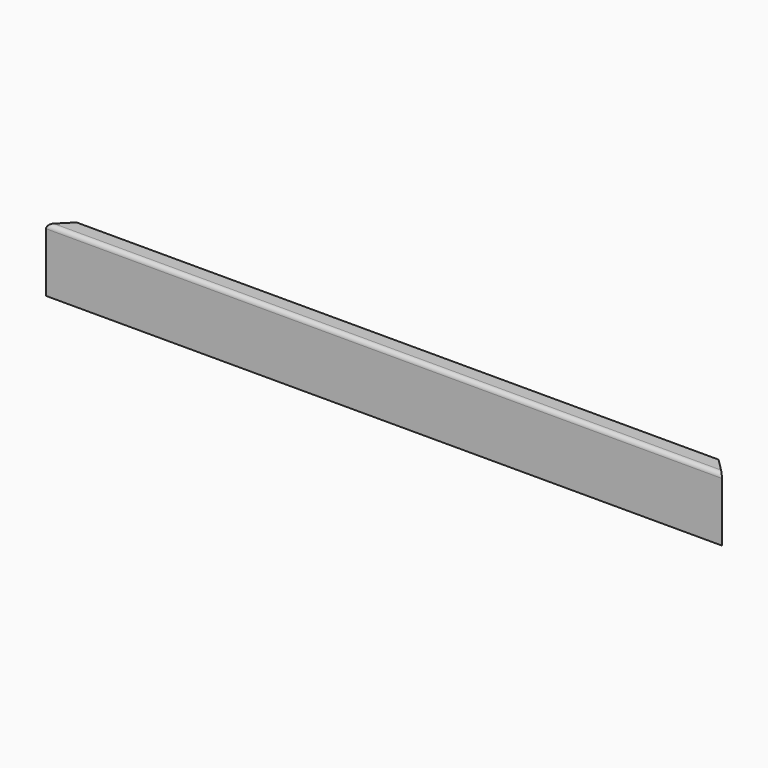
from build123d import *

# Parameters (mm, degrees)
F3_DEPTH  = 800
F4_SIZE   = 79.99999
F5_R      = 6
F6_DEPTH  = 50
F7_W      = 116
F7_H      = 90
F8_DEPTH  = 5
F9_R      = 10
F10_W     = 100
F10_H     = 100
F11_DEPTH = 20


# Not quite as in the source:
# - a fillet or chamfer is up to 0.001 mm smaller than in the source, because OpenCascade refuses the exact size


with BuildPart() as f3:
    # F2 (on Right) → F3 (new body, symmetric)
    with BuildSketch(Plane.YZ):
        Polygon((-40, 75), (-40, -75), (40, -75), (40, 15), (0, 15), (0, 75), align=None)
    extrude(amount=F3_DEPTH, both=True)

    # F4 (size 80 in the source; OpenCascade refuses exactly that, so slightly less here)
    f4_edges = [f3.edges().sort_by_distance(p)[0] for p in [
        (800, 40, -30),
        (-800, 40, -30),
    ]]
    chamfer(f4_edges, length=F4_SIZE)

    # F5 (on face) → F6 (cut)
    with BuildSketch(Plane(origin=(0, 40, 0), x_dir=(-1, 0, 0), z_dir=(0, 1, 0))):
        with Locations((-690, -45)):
            Circle(F5_R)
        with Locations((-670, -5)):
            Circle(F5_R)
        with Locations((670, -5)):
            Circle(F5_R)
        with Locations((690, -45)):
            Circle(F5_R)
    extrude(amount=-F6_DEPTH, mode=Mode.SUBTRACT)

    # F7 (on face) → F8 (cut)
    with BuildSketch(Plane(origin=(0, 40, 0), x_dir=(-1, 0, 0), z_dir=(0, 1, 0))):
        with Locations((-702, -30)):
            Rectangle(F7_W, F7_H)
        with Locations((702, -30)):
            Rectangle(F7_W, F7_H)
    extrude(amount=-F8_DEPTH, mode=Mode.SUBTRACT)

    # F9
    f9_edges = [f3.edges().sort_by_distance(p)[0] for p in [
        (0, -40, 75),
    ]]
    fillet(f9_edges, radius=F9_R)

    # F10 (on face) → F11 (cut)
    with BuildSketch(Plane(origin=(0, 0, -75), x_dir=(1, 0, 0), z_dir=(0, 0, -1))):
        with Locations((-710, -50)):
            Rectangle(F10_W, F10_H)
    extrude(amount=-F11_DEPTH, mode=Mode.SUBTRACT)


solid = f3.part
